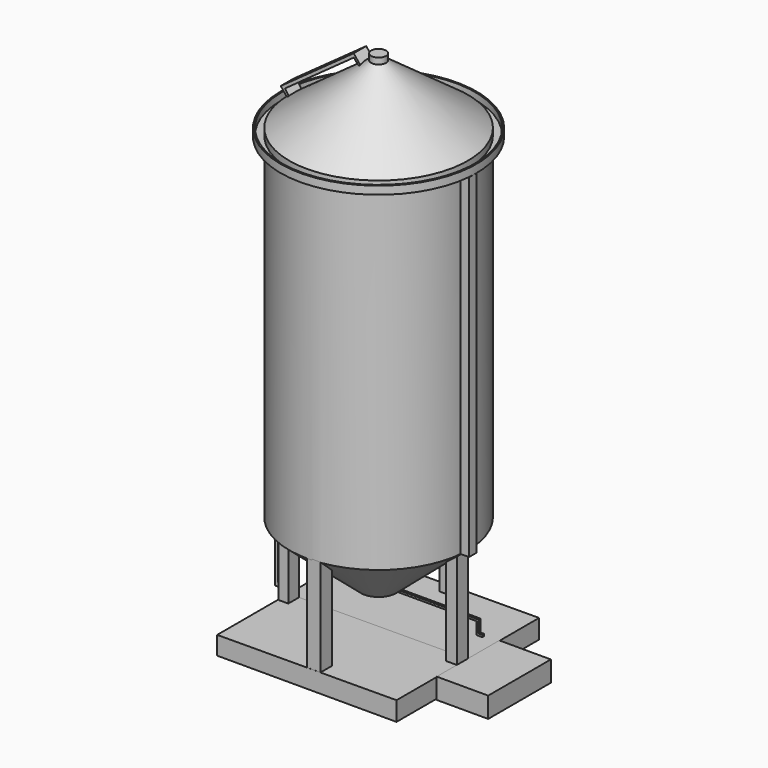
from build123d import *

# Parameters (mm, degrees)
F3_DEPTH  = 3.048
F5_DEPTH  = 4.318
F7_DEPTH  = 4.318
F9_DEPTH  = 0.762
F11_DEPTH = 28.829
F12_DEPTH = 28.956
F13_W     = 16.6921205819
F13_H     = 6.6633298993
F14_DEPTH = 12.7
F15_DEPTH = 12.7
F19_DEPTH = 2.54
F21_DEPTH = 2.54
F22_DEPTH = 5.08
F23_DEPTH = 2.54


# Not quite as in the source:
# - the program builds the solid bodies; features that only make, move or delete a surface that nothing else refers to are left out


with BuildPart() as f1:
    # F0 (on Front) → F1 (revolve)
    with BuildSketch(Plane.XZ):
        Polygon((-2.3954606149, 74.7646167874), (-28.9675891399, 55.4885827005), (-28.9675891399, 53.2673075795), (-31.3170477748, 53.2673075795), (-31.3170477748, 55.4885827005), (-31.7997783422, 55.4885827005), (-31.7997783422, 52.8993345797), (-28.9675891399, 52.8993345797), (-28.9675891399, -55.6848309934), (-5.7121798845, -75.5053013563), (0, -75.5053013563), (0, 76.7557322979), (-2.3954606149, 76.7557322979), align=None)
    revolve(axis=Axis((0, 0, 0.6252154708), (0, 0, -1)))

    # F2 (on Front) → F3 (join)
    with BuildSketch(Plane.XZ):
        Polygon((31.7770019174, -55.5002428591), (31.7770019174, 52.905689925), (28.998484835, 52.9252886772), (28.998484835, -55.5002428591), align=None)
    extrude(amount=F3_DEPTH)

    # F4 (on Front) → F5 (join)
    with BuildSketch(Plane.XZ):
        Polygon((28.9578214288, -88.7783765793), (28.9578214288, -55.7038187981), (25.253970176, -58.4993101656), (25.253970176, -88.7783765793), align=None)
    extrude(amount=F5_DEPTH)

    # F6 (on Right) → F7 (join)
    with BuildSketch(Plane.YZ):
        Polygon((-24.2134649307, -59.5846176147), (-28.9282295853, -55.377587676), (-28.9282295853, -88.8268202543), (-24.8995702714, -88.8268202543), (-24.2134649307, -88.8268202543), align=None)
        Polygon((28.9567187428, -89.0825837851), (28.9567187428, -55.8331161737), (24.6087126434, -58.902297169), (24.6087126434, -89.0825837851), align=None)
    extrude(amount=F7_DEPTH)

    # F8 (on Front) → F9 (join)
    with BuildSketch(Plane.XZ):
        Polygon((6.2913792208, -75.0306099653), (6.6843754612, -75.0306099653), (31.6898301244, -75.0306099653), (31.6898301244, -79.0014341474), (33.6215831339, -79.0014341474), (33.6215831339, -78.3609896898), (32.4000269175, -78.3609896898), (32.4000269175, -74.3909329176), (7.1138450876, -74.3909329176), align=None)
    extrude(amount=-F9_DEPTH)

    # F20 (on Front) → F21 (join)
    with BuildSketch(Plane.XZ):
        Polygon((-6.0486025177, 75.7997408509), (-29.6922810376, 58.7870106101), (-27.2098183632, 55.7047426701), (-26.6596407538, 56.2070166686), (-28.3279228477, 58.5255349164), (-6.0055375566, 74.587533009), (-3.9922085164, 72.2375285146), (-3.4829450306, 72.6527124643), align=None)
    extrude(amount=-F21_DEPTH)

    # F22 (add): a face of the model
    f22_faces = [f1.faces().sort_by_distance(p)[0] for p in [
        (-17.4845819472, 2.54, 66.7374198953),
    ]]
    extrude(f22_faces, amount=-F22_DEPTH)


with BuildPart() as f5:
    # F4 (on Front) → F5, piece 2 (new body)
    with BuildSketch(Plane.XZ):
        Polygon((-25.8202198893, -58.4993101656), (-28.9962254465, -55.7038187981), (-28.9962254465, -88.7783765793), (-25.8202198893, -88.7783765793), align=None)
    extrude(amount=F5_DEPTH)


with BuildPart() as f11:
    # F10 (on Front) → F11 (new body)
    with BuildSketch(Plane.XZ):
        Polygon((28.9828833193, -86.7293998599), (-29.1760452092, -86.9926735759), (-29.1760452092, -92.9283499718), (28.9828833193, -92.9283499718), align=None)
    extrude(amount=-F11_DEPTH)


with BuildPart() as f12:
    # F12 (new): a face of the model
    f12_faces = [f11.part.faces().sort_by_distance(p)[0] for p in [
        (0.113722427, 0, -89.8942173444),
    ]]
    extrude(f12_faces, amount=F12_DEPTH)


with BuildPart() as f14:
    # F13 (on Front) → F14 (new body)
    with BuildSketch(Plane.XZ):
        with Locations((37.3520161957, -89.9229906499)):
            Rectangle(F13_W, F13_H)
    extrude(amount=-F14_DEPTH)

    # F15 (add): a face of the model
    f15_faces = [f14.faces().sort_by_distance(p)[0] for p in [
        (37.3520161957, 0, -89.9229906499),
    ]]
    extrude(f15_faces, amount=F15_DEPTH)


with BuildPart() as f19:
    # F18 (on Front) → F19 (new body)
    with BuildSketch(Plane.XZ):
        Polygon((-31.5210707486, -84.4060778618), (-28.9624538273, -84.4060778618), (-28.9624538273, -83.1516385078), (-30.5430497974, -83.1516385078), (-30.5430497974, 48.9110127091), (-28.7834573537, 48.9110127091), (-28.7834573537, 50.1476339996), (-31.5210707486, 50.1476339996), align=None)
    extrude(amount=F19_DEPTH)


with BuildPart() as f23:
    # F23 (new): a face of the model
    f23_faces = [f19.part.faces().sort_by_distance(p)[0] for p in [
        (-30.9914355027, 0, -17.034232655),
    ]]
    extrude(f23_faces, amount=F23_DEPTH)


solid = Compound([f1.part, f5.part, f11.part, f12.part, f14.part, f19.part, f23.part])
